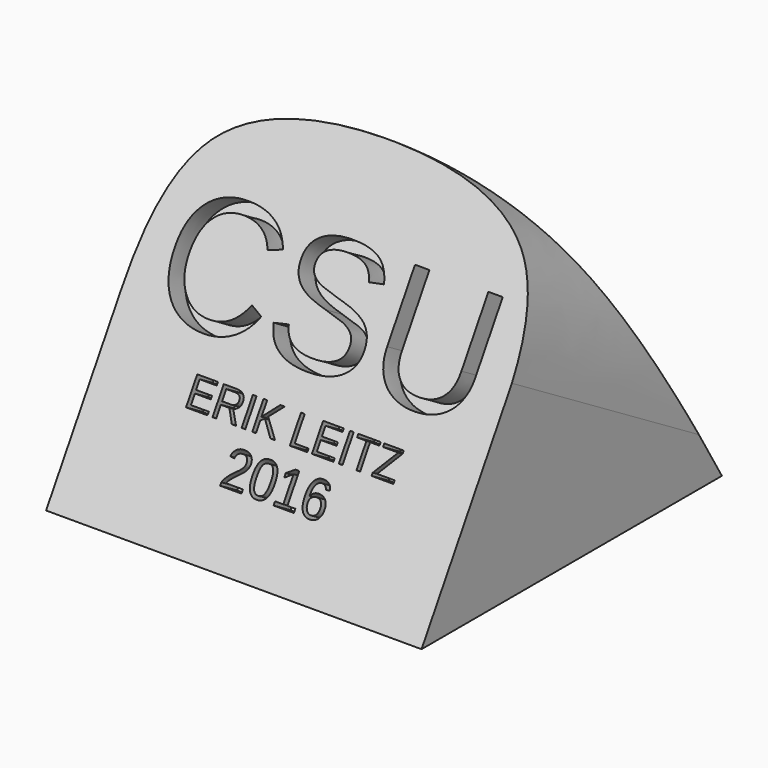
from build123d import *

# Parameters (mm, degrees)
F0_W           = 76.2
F0_H           = 76.2
F1_DEPTH       = 63.5
F3_DEPTH       = 76.201
F4_TEXT_SIZE   = 31.36150125
F5_DEPTH       = 5
F6_TEXT_SIZE   = 8.0619679971
F6_TEXT_SIZE_2 = 9.5317838714
F7_DEPTH       = 5
F9_DEPTH       = 65.3419609907
F10_TEXT_SIZE  = 7.6564119526
F11_DEPTH      = 5


# Not quite as in the source:
# - Text() gives the source's letters only with a copy of the font that has no kerning and outlines rounded to 1/6400 em; it was checked with that copy


with BuildPart() as f1:
    # F0 (on Top) → F1 (new body)
    with BuildSketch(Plane.XY):
        with Locations((-2.0151348621, 21.4075768084)):
            Rectangle(F0_W, F0_H)
    extrude(amount=F1_DEPTH)

    # F2 (on face) → F3 (cut, through all)
    with BuildSketch(Plane.YZ.offset(36.0848651379)):
        Polygon((-16.6924231916, 0), (21.4075768084, 63.5), (-16.6924231916, 63.5), align=None)
        Polygon((59.5075768084, 63.5), (21.4075768084, 63.5), (59.5075768084, 0), align=None)
    extrude(amount=-F3_DEPTH, mode=Mode.SUBTRACT)

    # F4 (on face) → F5 (cut)
    with BuildSketch(Plane(origin=(0, -12.273840582, 7.3643043492), x_dir=(1, 0, 0), z_dir=(0, -0.8574929257, 0.5144957554))):
        with Locations((-34.6425119787, 26.7064571381)):
            Text('CSU', F4_TEXT_SIZE, font='Arimo', text_align=(TextAlign.LEFT, TextAlign.BOTTOM))
    extrude(amount=-F5_DEPTH, mode=Mode.SUBTRACT)

    # F6 (on face) → F7 (cut)
    with BuildSketch(Plane(origin=(0, -12.273840582, 7.3643043492), x_dir=(1, 0, 0), z_dir=(0, -0.8574929257, 0.5144957554))):
        with Locations((-21.8615508638, 14.4530963153)):
            Text('ERIK LEITZ', F6_TEXT_SIZE, font='Arimo', text_align=(TextAlign.LEFT, TextAlign.BOTTOM))
        with Locations((-10.7225121847, 4.6636494808)):
            Text('2016', F6_TEXT_SIZE_2, font='Arimo', text_align=(TextAlign.LEFT, TextAlign.BOTTOM))
    extrude(amount=-F7_DEPTH, mode=Mode.SUBTRACT)

    # F8 (on face) → F9 (cut, through all)
    with BuildSketch(Plane(origin=(0, -12.273840582, 7.3643043492), x_dir=(1, 0, 0), z_dir=(0, -0.8574929257, 0.5144957554))):
        with BuildLine():
            Line((-40.1151348621, 65.4649081847), (-40.1151348621, 28.4383636524))
            add(Edge.make_bspline(
                [(-40.1151348621, 28.4383636524), (-40.1151348621, 38.3890179374), (-37.6425909687, 60.8001490816), (-14.3002056597, 65.3203412589), (-2.0151348621, 65.4649081847)],
                knots=[0, 0, 0, 0, 0.241102538, 0.4980768722, 0.4980768722, 0.4980768722, 0.4980768722], degree=3))
            Line((-2.0151348621, 65.4649081847), (-40.1151348621, 65.4649081847))
        make_face()
        with BuildLine():
            Line((36.0848651379, 65.4649081847), (0.3597500725, 65.4649081847))
            add(Edge.make_bspline(
                [(0.3597500725, 65.4649081847), (11.9601136428, 65.3249810378), (32.1624576493, 61.373589625), (35.7606188064, 43.9268264942), (36.0848651379, 35.963672106)],
                knots=[0.5146263809, 0.5146263809, 0.5146263809, 0.5146263809, 0.7571698018, 0.9421654114, 0.9421654114, 0.9421654114, 0.9421654114], degree=3))
            Line((36.0848651379, 35.963672106), (36.0848651379, 65.4649081847))
        make_face()
    extrude(amount=-F9_DEPTH, mode=Mode.SUBTRACT)

    # F10 (on face) → F11 (cut)
    with BuildSketch(Plane(origin=(0, 43.7555711827, 26.2533427096), x_dir=(-1, 0, 0), z_dir=(0, 0.8574929257, 0.5144957554))):
        with Locations((-36.0848651379, -24.7660498916)):
            Text('GOOD LUCK! -EMILY', F10_TEXT_SIZE, font='Arimo', text_align=(TextAlign.LEFT, TextAlign.BOTTOM))
    extrude(amount=-F11_DEPTH, mode=Mode.SUBTRACT)


solid = f1.part
